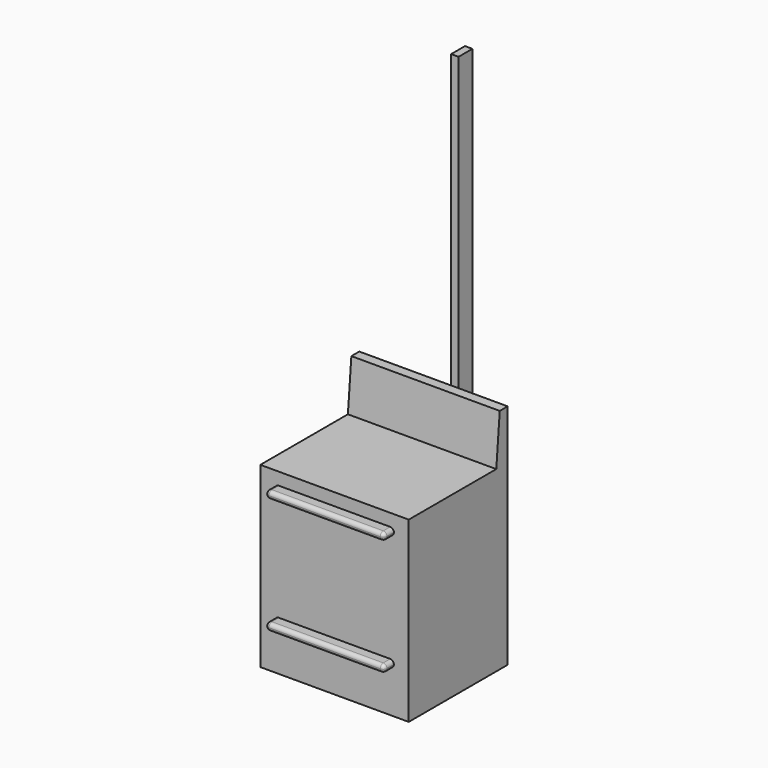
from build123d import *

# Parameters (mm, degrees)
F1_DEPTH  = 381
F2_W      = 63.5
F2_H      = 38.1
F3_DEPTH  = 304.8
F4_R      = 19.04999
F5_W      = 38.1
F5_H      = 88.9
F6_DEPTH  = 838.2
F7_DEPTH  = 2590.8
F8_DEPTH  = 939.8
F9_DEPTH  = 1011.30608
F10_DEPTH = 698.5


# Not quite as in the source:
# - a fillet or chamfer is up to 0.001 mm smaller than in the source, because OpenCascade refuses the exact size


with BuildPart() as f1:
    # F0 (on Right) → F1 (new body, symmetric)
    with BuildSketch(Plane.YZ):
        Polygon((-635, 0), (0, 0), (0, 1168.4), (-50.8, 1168.4), (-73.0221205356, 914.4), (-635, 914.4), align=None)
    extrude(amount=F1_DEPTH, both=True)

    # F2 (on Right) → F3 (join, symmetric)
    with BuildSketch(Plane.YZ):
        with Locations((-666.75, 831.85)):
            Rectangle(F2_W, F2_H)
        with Locations((-666.75, 234.95)):
            Rectangle(F2_W, F2_H)
    extrude(amount=F3_DEPTH, both=True)

    # F4 (radius 19.05 in the source; OpenCascade refuses exactly that, so slightly less here)
    f4_edges = [f1.edges().sort_by_distance(p)[0] for p in [
        (0, -698.5, 850.9),
        (0, -698.5, 812.8),
        (-304.8, -698.5, 831.85),
        (304.8, -698.5, 831.85),
        (304.8, -666.75, 850.9),
        (304.8, -666.75, 812.8),
        (-304.8, -666.75, 850.9),
        (-304.8, -666.75, 812.8),
        (-304.8, -666.75, 254),
        (-304.8, -666.75, 215.9),
        (0, -698.5, 215.9),
        (-304.8, -698.5, 234.95),
        (304.8, -698.5, 234.95),
        (0, -698.5, 254),
        (304.8, -666.75, 254),
        (304.8, -666.75, 215.9),
    ]]
    fillet(f4_edges, radius=F4_R)


with BuildPart() as f6:
    # F5 (on Top) → F6 (new body)
    with BuildSketch(Plane.XY):
        with Locations((19.05, 157.7875594588)):
            Rectangle(F5_W, F5_H)
    extrude(amount=F6_DEPTH)


with BuildPart() as f7:
    # F5 (on Top) → F7 (new body)
    with BuildSketch(Plane.XY):
        with Locations((19.05, 157.7875594588)):
            Rectangle(F5_W, F5_H)
    extrude(amount=F7_DEPTH)


with BuildPart() as f8:
    # F5 (on Top) → F8 (new body)
    with BuildSketch(Plane.XY):
        with Locations((19.05, 157.7875594588)):
            Rectangle(F5_W, F5_H)
    extrude(amount=F8_DEPTH)


with BuildPart() as f9:
    # F5 (on Top) → F9 (new body)
    with BuildSketch(Plane.XY):
        with Locations((19.05, 157.7875594588)):
            Rectangle(F5_W, F5_H)
    extrude(amount=F9_DEPTH)


with BuildPart() as f10:
    # F5 (on Top) → F10 (new body)
    with BuildSketch(Plane.XY):
        with Locations((19.05, 157.7875594588)):
            Rectangle(F5_W, F5_H)
    extrude(amount=F10_DEPTH)


solid = Compound([f1.part, f6.part, f7.part, f8.part, f9.part, f10.part])
